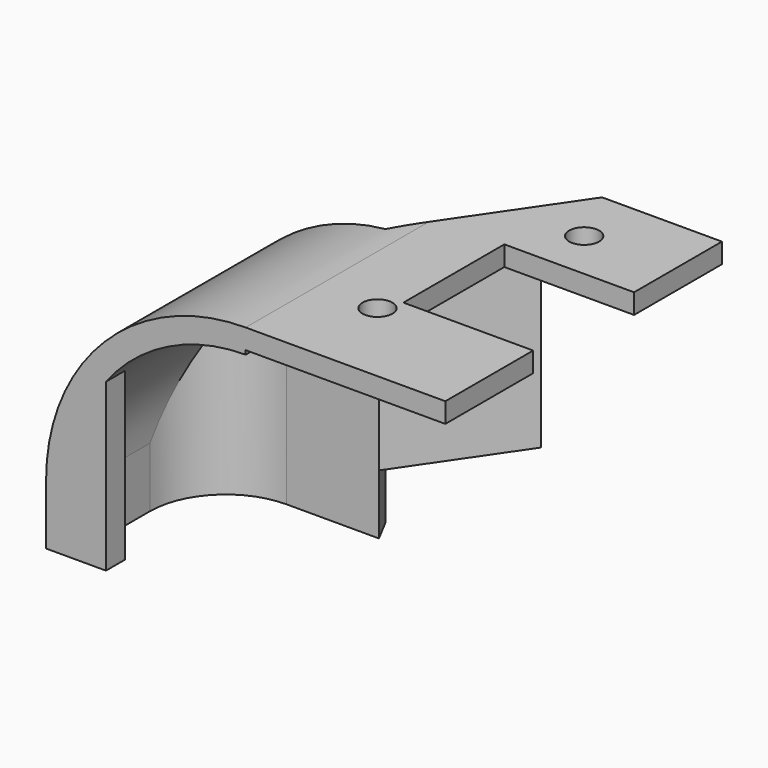
from build123d import *

# Parameters (mm, degrees)
F0_R      = 1.5
F1_DEPTH  = 2
F2_DEPTH  = 24
F4_DEPTH  = 25
F5_R      = 1.5
F6_DEPTH  = 24
F8_DEPTH  = 20
F10_DEPTH = 25
F11_DEPTH = 6


# Not quite as in the source:
# - a feature names something its author has since deleted; it is built from what else it names


with BuildPart() as f1:
    # F0 (on Top) → F1 (new body)
    with BuildSketch(Plane.XY):
        with BuildLine():
            Line((-20, -17.6375247538), (20, -17.6375247538))
            Line((20, -17.6375247538), (20, -6.6375247538))
            Line((20, -6.6375247538), (7, -6.6375247538))
            Line((7, -6.6375247538), (7, 6))
            Line((7, 6), (20, 6))
            Line((20, 6), (20, 17))
            Line((20, 17), (8, 17))
            Line((8, 17), (-2, 2.3624752462))
            Line((-2, 2.3624752462), (-10, 2.3624752462))
            ThreePointArc((-10, 2.3624752462), (-17.0710678119, -0.5664569419), (-20, -7.6375247538))
            Line((-20, -7.6375247538), (-20, -17.6375247538))
        make_face()
        with Locations((6, -8.6375247538)):
            Circle(F0_R, mode=Mode.SUBTRACT)
        with Locations((11, 11)):
            Circle(F0_R, mode=Mode.SUBTRACT)
    extrude(amount=F1_DEPTH)

    # F2 (add): a face of the model
    f2_faces = [f1.faces().sort_by_distance(p)[0] for p in [
        (0.9940051369, -4.5309976768, 0),
    ]]
    extrude(f2_faces, amount=F2_DEPTH)

    # F3 (on face) → F4 (cut)
    with BuildSketch(Plane.XZ.offset(17.6375247538)):
        with BuildLine():
            Line((-20, -11), (-20, -18))
            ThreePointArc((-20, -18), (-14.1421356237, -3.8578643763), (0, 2))
            Line((0, 2), (-7, 2))
            Line((-7, 2), (-20, 2))
            Line((-20, 2), (-20, -11))
        make_face()
    extrude(amount=-F4_DEPTH, mode=Mode.SUBTRACT)

    # F5 (on face) → F6 (cut)
    with BuildSketch(Plane(origin=(0, 0, -24), x_dir=(1, 0, 0), z_dir=(0, 0, -1))):
        with BuildLine():
            Line((20, 17.6375247538), (-14, 17.6375247538))
            Line((-14, 17.6375247538), (-14, 15.2375247538))
            Line((-14, 15.2375247538), (-17.6, 15.2375247538))
            Line((-17.6, 15.2375247538), (-17.6, 7.6375247538))
            ThreePointArc((-17.6, 7.6375247538), (-15.374011537, 2.2635132168), (-10, 0.0375247538))
            Line((-10, 0.0375247538), (-0.7330154527, 0.0375247538))
            Line((-0.7330154527, 0.0375247538), (6.7509134438, -10.9170946941))
            Line((6.7509134438, -10.9170946941), (4.7692207252, -12.2709388392))
            Line((4.7692207252, -12.2709388392), (8, -17))
            Line((8, -17), (20, -17))
            Line((20, -17), (20, -6))
            Line((20, -6), (7, -6))
            Line((7, -6), (7, 6.6375247538))
            Line((7, 6.6375247538), (20, 6.6375247538))
            Line((20, 6.6375247538), (20, 17.6375247538))
        make_face()
        with Locations((11, -11)):
            Circle(F5_R, mode=Mode.SUBTRACT)
        with Locations((6, 8.6375247538)):
            Circle(F5_R, mode=Mode.SUBTRACT)
    extrude(amount=-F6_DEPTH, mode=Mode.SUBTRACT)

    # F7 (on face) → F8 (join)
    with BuildSketch(Plane.XZ.offset(17.6375247538)):
        with BuildLine():
            Line((0, -0.4), (0, 2))
            ThreePointArc((0, 2), (-14.1421356237, -3.8578643763), (-20, -18))
            Line((-20, -18), (-17.6, -18))
            ThreePointArc((-17.6, -18), (-12.4450793489, -5.5549206511), (0, -0.4))
        make_face()
    extrude(amount=-F8_DEPTH)

    # F9 (on face) → F10 (cut)
    with BuildSketch(Plane(origin=(0, 0, -24), x_dir=(1, 0, 0), z_dir=(0, 0, -1))):
        with BuildLine():
            ThreePointArc((-25, 7.6375247538), (-20.6066017178, -2.969076964), (-10, -7.3624752462))
            Line((-10, -7.3624752462), (-10, -2.3624752462))
            ThreePointArc((-10, -2.3624752462), (-17.0710678119, 0.5664569419), (-20, 7.6375247538))
            Line((-20, 7.6375247538), (-25, 7.6375247538))
        make_face()
    extrude(amount=-F10_DEPTH, mode=Mode.SUBTRACT)

    # F5 (on face) → F11 (cut)
    with BuildSketch(Plane(origin=(0, 0, -24), x_dir=(1, 0, 0), z_dir=(0, 0, -1))):
        Polygon((-0.7330154527, 0.0375247538), (-2, -2.3624752462), (4.7692207252, -12.2709388392), (6.7509134438, -10.9170946941), align=None)
    extrude(amount=-F11_DEPTH, mode=Mode.SUBTRACT)


solid = f1.part
